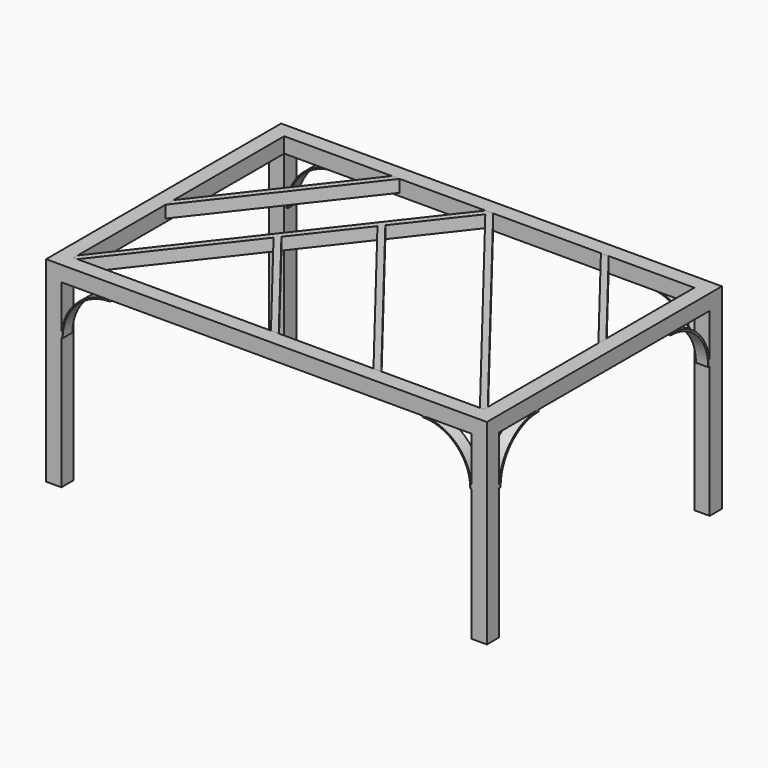
from build123d import *

# Parameters (mm, degrees)
F0_W      = 914.4
F0_H      = 609.6
F1_DEPTH  = 15.875
F2_W      = 850.9
F2_H      = 546.1
F3_DEPTH  = 31.751
F5_DEPTH  = 25.4
F6_W      = 31.75
F6_H      = 31.75
F7_DEPTH  = 374.65
F9_DEPTH  = 25.4
F12_DEPTH = 25.4


# Not quite as in the source:
# - a feature of the source that left no trace in its solid (it failed there, or was rolled back) is left out
# - a feature names something its author has since deleted; it is built from what else it names


with BuildPart() as f1:
    # F0 (on Top) → F1 (new body, symmetric)
    with BuildSketch(Plane.XY):
        Rectangle(F0_W, F0_H)
    extrude(amount=F1_DEPTH, both=True)

    # F2 (on face) → F3 (cut, through all)
    with BuildSketch(Plane.XY.offset(15.875)):
        Rectangle(F2_W, F2_H)
    extrude(amount=-F3_DEPTH, mode=Mode.SUBTRACT)

    # F6 (on face) → F7 (join)
    with BuildSketch(Plane(origin=(0, 0, -15.875), x_dir=(1, 0, 0), z_dir=(0, 0, -1))):
        with Locations((-441.325, 288.925)):
            Rectangle(F6_W, F6_H)
        with Locations((-441.325, -288.925)):
            Rectangle(F6_W, F6_H)
        with Locations((441.325, 288.925)):
            Rectangle(F6_W, F6_H)
        with Locations((441.325, -288.925)):
            Rectangle(F6_W, F6_H)
    extrude(amount=F7_DEPTH)


with BuildPart() as f5:
    # F4 (on face) → F5 (new body)
    with BuildSketch(Plane.XY.offset(15.875)):
        Polygon((-8.0496105111, 273.05), (-425.45, -262.7176641201), (-425.45, -273.05), (-417.4003894889, -273.05), (-216.7498052556, -15.4985038199), (-208.7001947444, -5.16616794), (-110.3873052556, 121.0264961801), (-102.3376947444, 131.35883206), (0, 262.7176641201), align=None)
        Polygon((8.0496105111, 273.05), (-8.0496105111, 273.05), (0, 262.7176641201), (417.4003894889, -273.05), (425.45, -273.05), (425.45, -262.7176641201), align=None)
        Polygon((212.725, -273.05), (-102.3376947444, 131.35883206), (-110.3873052556, 121.0264961801), (196.6257789778, -273.05), align=None)
        Polygon((-208.7001947444, -5.16616794), (-216.7498052556, -15.4985038199), (-16.0992210222, -273.05), (0, -273.05), align=None)
    extrude(amount=-F5_DEPTH)


with BuildPart() as f5b:
    # F4 (on face) → F5, piece 2 (new body)
    with BuildSketch(Plane.XY.offset(15.875)):
        Polygon((231.5507789778, 273.05), (425.45, 24.1644327177), (425.45, 44.8291044776), (247.65, 273.05), align=None)
    extrude(amount=-F5_DEPTH)


with BuildPart() as f5c:
    # F4 (on face) → F5, piece 3 (new body)
    with BuildSketch(Plane.XY.offset(15.875)):
        Polygon((-425.45, -13.8320968378), (-425.45, -34.4967685977), (-185.8496105111, 273.05), (-201.9488315334, 273.05), align=None)
    extrude(amount=-F5_DEPTH)


with BuildPart() as f9:
    # F8 (on face) → F9 (new body)
    with BuildSketch(Plane.XZ.offset(304.8)):
        with BuildLine():
            Line((-323.85, -18.415), (-323.85, -15.875))
            ThreePointArc((-323.85, -15.875), (-395.6920489686, -45.6329510314), (-425.45, -117.475))
            Line((-425.45, -117.475), (-422.91, -117.475))
            ThreePointArc((-422.91, -117.475), (-393.8959977443, -47.4290022557), (-323.85, -18.415))
        make_face()
    extrude(amount=-F9_DEPTH)


with BuildPart() as f9b:
    # F8 (on face) → F9, piece 2 (new body)
    with BuildSketch(Plane.XZ.offset(304.8)):
        with BuildLine():
            Line((323.85, -15.875), (323.85, -18.415))
            ThreePointArc((323.85, -18.415), (393.8959977443, -47.4290022557), (422.91, -117.475))
            Line((422.91, -117.475), (425.45, -117.475))
            ThreePointArc((425.45, -117.475), (395.6920489686, -45.6329510314), (323.85, -15.875))
        make_face()
    extrude(amount=-F9_DEPTH)


with BuildPart() as f10_1:
    # F10: instance of F9
    add(f9.part.mirror(Plane.XZ))


with BuildPart() as f10_2:
    # F10: instance of F9b
    add(f9b.part.mirror(Plane.XZ))


with BuildPart() as f12:
    # F11 (on face) → F12 (new body)
    with BuildSketch(Plane.YZ.offset(457.2)):
        with BuildLine():
            ThreePointArc((273.05, -117.475), (243.2920489686, -45.6329510314), (171.45, -15.875))
            Line((171.45, -15.875), (171.45, -19.685))
            ThreePointArc((171.45, -19.685), (240.5979721322, -48.3270278678), (269.24, -117.475))
            Line((269.24, -117.475), (273.05, -117.475))
        make_face()
    extrude(amount=-F12_DEPTH)


with BuildPart() as f12b:
    # F11 (on face) → F12, piece 2 (new body)
    with BuildSketch(Plane.YZ.offset(457.2)):
        with BuildLine():
            ThreePointArc((-269.24, -117.475), (-240.5979721322, -48.3270278678), (-171.45, -19.685))
            Line((-171.45, -19.685), (-171.45, -15.875))
            ThreePointArc((-171.45, -15.875), (-243.2920489686, -45.6329510314), (-273.05, -117.475))
            Line((-273.05, -117.475), (-269.24, -117.475))
        make_face()
    extrude(amount=-F12_DEPTH)


solid = Compound([f1.part, f5.part, f5b.part, f5c.part, f9.part, f9b.part, f10_1.part, f10_2.part, f12.part, f12b.part])
